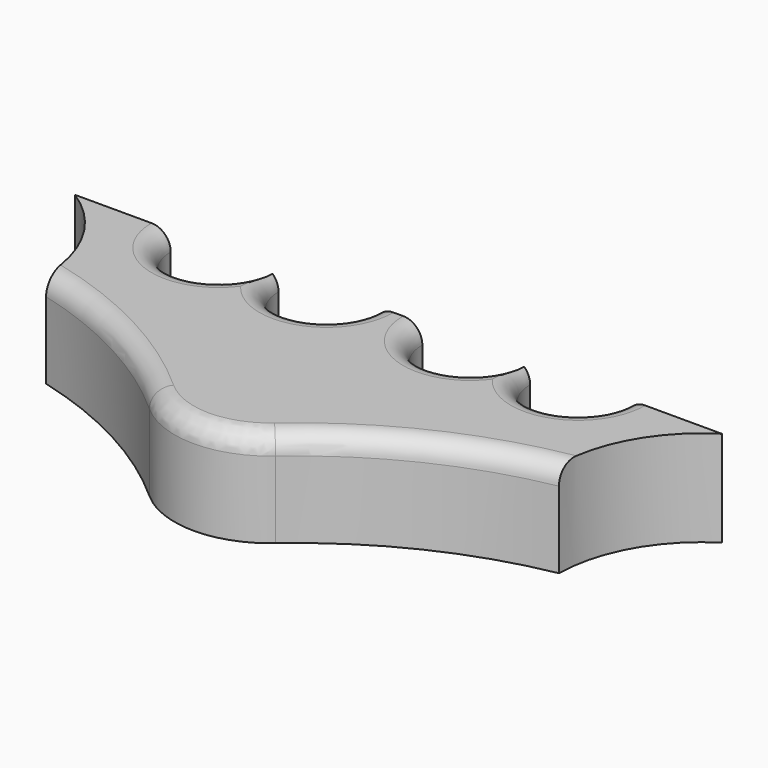
from build123d import *

# Parameters (mm, degrees)
F1_DEPTH    = 25.4
F2_R        = 25.4
F3_T2_ANGLE = 294.7758439205
F3_T4_ANGLE = 294.7758439205
F3_T6_ANGLE = 294.7758439205
F3_T8_ANGLE = 294.7758439205
F4_R        = 5.08


# Not quite as in the source:
# - a fillet or chamfer that OpenCascade refuses, or shapes differently, is made with other operations: its cross-section is extruded or revolved along the edge and cut away or added


with BuildPart() as f1:
    # F0 (on Top) → F1 (new body)
    with BuildSketch(Plane.XY):
        with BuildLine():
            Line((37.1146484218, 92.3934370832), (11.7146484218, 92.3934370832))
            ThreePointArc((11.7146484218, 92.3934370832), (24.640162726, 78.7783250935), (29.4946484218, 60.6434370832))
            ThreePointArc((29.4946484218, 60.6434370832), (65.749840409, 44.0578596931), (94.2646484218, 16.1934370832))
            ThreePointArc((94.2646484218, 16.1934370832), (125.6004493922, 45.1771555306), (165.3846484218, 60.6434370832))
            ThreePointArc((165.3846484218, 60.6434370832), (170.2391341176, 78.7783250935), (183.1646484218, 92.3934370832))
            Line((183.1646484218, 92.3934370832), (157.7646484218, 92.3934370832))
            ThreePointArc((157.7646484218, 92.3934370832), (145.0646484218, 79.6934370832), (132.3646484218, 92.3934370832))
            Line((132.3646484218, 92.3934370832), (129.1896484218, 92.3934370832))
            ThreePointArc((129.1896484218, 92.3934370832), (116.4896484218, 79.6934370832), (103.7896484218, 92.3934370832))
            Line((103.7896484218, 92.3934370832), (91.0896484218, 92.3934370832))
            ThreePointArc((91.0896484218, 92.3934370832), (78.3896484218, 79.6934370832), (65.6896484218, 92.3934370832))
            Line((65.6896484218, 92.3934370832), (62.5146484218, 92.3934370832))
            ThreePointArc((62.5146484218, 92.3934370832), (49.8146484218, 79.6934370832), (37.1146484218, 92.3934370832))
        make_face()
    extrude(amount=F1_DEPTH)

    # F2
    f2_edges = [f1.edges().sort_by_distance(p)[0] for p in [
        (94.264648, 16.193437, 12.7),
    ]]
    fillet(f2_edges, radius=F2_R)

    # F3: fillet of radius 5.08 on 4 edges, made by hand

    # F3_s1 → F3_t2 (revolve, cut)
    with BuildSketch(Plane(origin=(-6.5992867665, 4.2223803326, 0), x_dir=(0, 0, 1), z_dir=(-0.8423388046, 0.5389483633, 0))):
        with BuildLine():
            ThreePointArc((25.4, 122.4541005786), (23.9121024484, 118.8619981302), (20.32, 117.3741005786))
            Line((20.32, 117.3741005786), (25.4, 117.3741005786))
            Line((25.4, 117.3741005786), (25.4, 122.4541005786))
        make_face()
    revolve(axis=Axis((49.8146484218, 92.3934370832, 25.4), (0, 0, -1)), revolution_arc=F3_T2_ANGLE, mode=Mode.SUBTRACT)

    # F3_s3 → F3_t4 (revolve, cut)
    with BuildSketch(Plane(origin=(40.7089368011, -26.0465441486, 0), x_dir=(0, 0, 1), z_dir=(-0.8423388046, 0.5389483633, 0))):
        with BuildLine():
            ThreePointArc((25.4, 158.3884827026), (23.9121024484, 154.7963802542), (20.32, 153.3084827026))
            Line((20.32, 153.3084827026), (25.4, 153.3084827026))
            Line((25.4, 153.3084827026), (25.4, 158.3884827026))
        make_face()
    revolve(axis=Axis((116.4896484218, 92.3934370832, 25.4), (0, 0, -1)), revolution_arc=F3_T4_ANGLE, mode=Mode.SUBTRACT)

    # F3_s5 → F3_t6 (revolve, cut)
    with BuildSketch(Plane(origin=(60.9838897586, -39.0189403548, 0), x_dir=(0, 0, 1), z_dir=(-0.8423388046, 0.5389483633, 0))):
        with BuildLine():
            ThreePointArc((25.4, 173.7889321843), (23.9121024484, 170.1968297359), (20.32, 168.7089321843))
            Line((20.32, 168.7089321843), (25.4, 168.7089321843))
            Line((25.4, 168.7089321843), (25.4, 173.7889321843))
        make_face()
    revolve(axis=Axis((145.0646484218, 92.3934370832, 25.4), (0, 0, -1)), revolution_arc=F3_T6_ANGLE, mode=Mode.SUBTRACT)

    # F3_s7 → F3_t8 (revolve, cut)
    with BuildSketch(Plane(origin=(13.6756661911, -8.7500158736, 0), x_dir=(0, 0, 1), z_dir=(-0.8423388046, 0.5389483633, 0))):
        with BuildLine():
            ThreePointArc((25.4, 137.8545500603), (23.9121024484, 134.2624476119), (20.32, 132.7745500603))
            Line((20.32, 132.7745500603), (25.4, 132.7745500603))
            Line((25.4, 132.7745500603), (25.4, 137.8545500603))
        make_face()
    revolve(axis=Axis((78.3896484218, 92.3934370832, 25.4), (0, 0, -1)), revolution_arc=F3_T8_ANGLE, mode=Mode.SUBTRACT)

    # F4
    f4_edges = [f1.edges().sort_by_distance(p)[0] for p in [
        (94.329479, 28.280902, 25.4),
    ]]
    fillet(f4_edges, radius=F4_R)


with BuildPart() as f5_1:
    # F5: copy of F1
    add(f1.part)


with BuildPart() as f6_1:
    # F6: copy of F5_1
    add(f5_1.part.moved(Location((0, 0, 50.8))))


solid = f1.part
